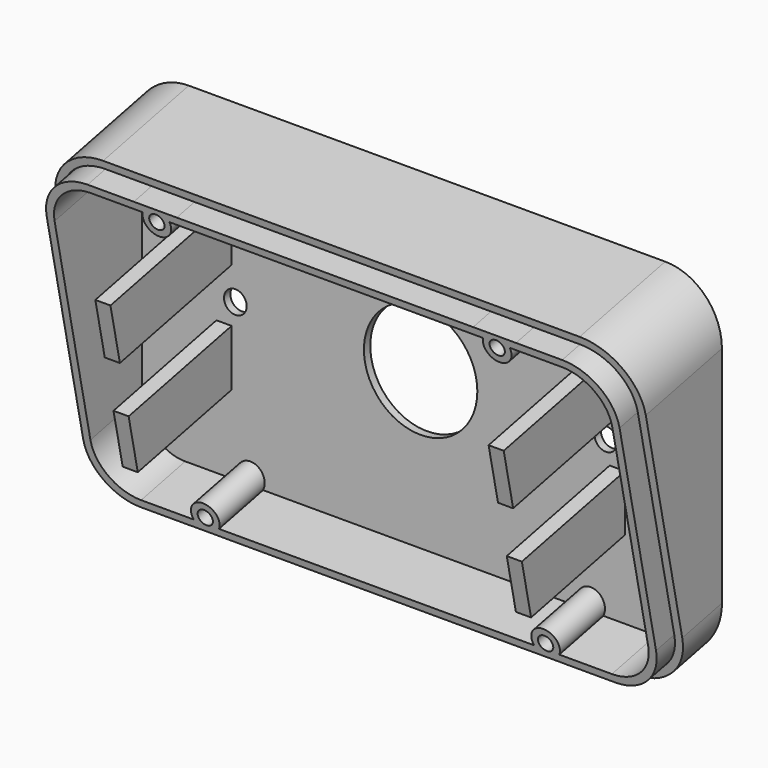
from build123d import *

# Parameters (mm, degrees)
F4_REACH  = 208.024207
F5_T      = -2.1
F6_R      = 15
F6_R_2    = 3
F7_DEPTH  = 25
F10_REACH = 207.704957
F14_W     = 4
F14_H     = 14.565263
F14_H_2   = 15
F15_REACH = 58.597972
F16_R     = 3.75
F17_REACH = 44.386615
F18_R     = 2
F19_REACH = 39.436868
F20_W     = 11.335485
F20_H     = 8.524533
F20_W_2   = 8.857343
F20_H_2   = 2.930835
F21_DEPTH = 25


with BuildPart() as f4:
    f4_end = Plane(origin=(0, 0, 0), x_dir=(0, 0, -1), z_dir=(0, -1, 0))
    # F3 (on line) → F4 (new body, up to a plane its end follows)
    with BuildSketch(Plane(origin=(0, -19.135318, -4.067337), x_dir=(-1, 0, 0), z_dir=(0, 0.978148, 0.207912))):
        with BuildLine():
            Line((63, 44), (-63, 44))
            ThreePointArc((-63, 44), (-73.606602, 39.606602), (-78, 29))
            Line((-78, 29), (-78, -29))
            ThreePointArc((-78, -29), (-73.606602, -39.606602), (-63, -44))
            Line((-63, -44), (63, -44))
            ThreePointArc((63, -44), (73.606602, -39.606602), (78, -29))
            Line((78, -29), (78, 29))
            ThreePointArc((78, 29), (73.606602, 39.606602), (63, 44))
        make_face()
    f4_long = extrude(amount=F4_REACH, mode=Mode.PRIVATE)
    add(split(f4_long, bisect_by=f4_end, keep=Keep.TOP, mode=Mode.PRIVATE))

    # F5
    f5_openings = [f4.faces().sort_by_distance(p)[0] for p in [
        (0, -19.135318, -4.067337),
    ]]
    offset(amount=F5_T, openings=f5_openings, kind=Kind.INTERSECTION)

    # F6 (on Front) → F7 (cut)
    with BuildSketch(Plane.XZ):
        Circle(F6_R)
        with Locations((-49, 0)):
            Circle(F6_R_2)
        with Locations((49, 0)):
            Circle(F6_R_2)
    extrude(amount=F7_DEPTH, mode=Mode.SUBTRACT)

    f10_end = Plane(origin=(0, 0, 0), x_dir=(0, 0, -1), z_dir=(0, -1, 0))
    # F9 (on offset) → F10 (join, up to a plane its end follows)
    with BuildSketch(Plane(origin=(0, -25.004204, -5.314808), x_dir=(-1, 0, 0), z_dir=(0, 0.978148, 0.207912))):
        with BuildLine():
            Line((62.75, 41.933544), (-62.75, 41.933544))
            ThreePointArc((-62.75, 41.933544), (-71.942388, 38.125932), (-75.75, 28.933544))
            Line((-75.75, 28.933544), (-75.75, -29.066456))
            ThreePointArc((-75.75, -29.066456), (-71.942388, -38.258845), (-62.75, -42.066456))
            Line((-62.75, -42.066456), (62.75, -42.066456))
            ThreePointArc((62.75, -42.066456), (71.942388, -38.258845), (75.75, -29.066456))
            Line((75.75, -29.066456), (75.75, 28.933544))
            ThreePointArc((75.75, 28.933544), (71.942388, 38.125932), (62.75, 41.933544))
        make_face()
        with BuildLine():
            ThreePointArc((-73.75, 28.433544), (-70.381728, 36.565272), (-62.25, 39.933544))
            Line((-62.25, 39.933544), (62.25, 39.933544))
            ThreePointArc((62.25, 39.933544), (70.381728, 36.565272), (73.75, 28.433544))
            Line((73.75, 28.433544), (73.75, -28.566456))
            ThreePointArc((73.75, -28.566456), (70.381728, -36.698184), (62.25, -40.066456))
            Line((62.25, -40.066456), (-62.25, -40.066456))
            ThreePointArc((-62.25, -40.066456), (-70.381728, -36.698184), (-73.75, -28.566456))
            Line((-73.75, -28.566456), (-73.75, 28.433544))
        make_face(mode=Mode.SUBTRACT)
    f10_long = extrude(amount=F10_REACH, mode=Mode.PRIVATE)
    add(split(f10_long, bisect_by=f10_end, keep=Keep.TOP, mode=Mode.PRIVATE))

    f15_end = Plane(origin=(0, 0, 0), x_dir=(0, 0, -1), z_dir=(0, -1, 0))
    # F14 (on offset) → F15 (join, up to a plane its end follows)
    with BuildSketch(Plane(origin=(0, -37.231049, -7.913704), x_dir=(-1, 0, 0), z_dir=(0, 0.978148, 0.207912))):
        with Locations((52, -12.588934)):
            Rectangle(F14_W, F14_H)
        with Locations((52, 16.074831)):
            Rectangle(F14_W, F14_H_2)
        with Locations((-52, 16.074831)):
            Rectangle(F14_W, F14_H_2)
        with Locations((-52, -12.588934)):
            Rectangle(F14_W, F14_H)
    f15_long = extrude(amount=F15_REACH, mode=Mode.PRIVATE)
    add(split(f15_long, bisect_by=f15_end, keep=Keep.TOP, mode=Mode.PRIVATE))

    f17_end = Plane(origin=(0, 0, 0), x_dir=(0, 0, -1), z_dir=(0, -1, 0))
    # F16 (on offset) → F17 (join, up to a plane its end follows)
    with BuildSketch(Plane(origin=(0, -25.004204, -5.314808), x_dir=(-1, 0, 0), z_dir=(0, 0.978148, 0.207912))):
        with Locations((45, 38.65889)):
            Circle(F16_R)
        with Locations((-45, 38.65889)):
            Circle(F16_R)
        with Locations((45, -38.34111)):
            Circle(F16_R)
        with Locations((-45, -38.34111)):
            Circle(F16_R)
    f17_long = extrude(amount=F17_REACH, mode=Mode.PRIVATE)
    add(split(f17_long, bisect_by=f17_end, keep=Keep.TOP, mode=Mode.PRIVATE))

    f19_end = Plane(origin=(0, 0, 0), x_dir=(0, 0, -1), z_dir=(0, -1, 0))
    # F18 (on offset) → F19 (cut, up to a plane its end follows)
    with BuildSketch(Plane(origin=(0, -25.004204, -5.314808), x_dir=(-1, 0, 0), z_dir=(0, 0.978148, 0.207912))):
        with Locations((45, 38.65889)):
            Circle(F18_R)
        with Locations((-45, 38.65889)):
            Circle(F18_R)
        with Locations((45, -38.34111)):
            Circle(F18_R)
        with Locations((-45, -38.34111)):
            Circle(F18_R)
    f19_long = extrude(amount=F19_REACH, mode=Mode.PRIVATE)
    add(split(f19_long, bisect_by=f19_end, keep=Keep.TOP, mode=Mode.PRIVATE), mode=Mode.SUBTRACT)

    # F20 (on line) → F21 (cut)
    with BuildSketch(Plane(origin=(0, -19.135318, -4.067337), x_dir=(-1, 0, 0), z_dir=(0, 0.978148, 0.207912))):
        with Locations((44.866957, 46.19581)):
            Rectangle(F20_W, F20_H)
        with Locations((-44.866957, 46.19581)):
            Rectangle(F20_W, F20_H)
        with Locations((44.735221, -43.516963)):
            Rectangle(F20_W_2, F20_H_2)
        with Locations((-44.735221, -43.516963)):
            Rectangle(F20_W_2, F20_H_2)
    extrude(amount=-F21_DEPTH, mode=Mode.SUBTRACT)


solid = f4.part
